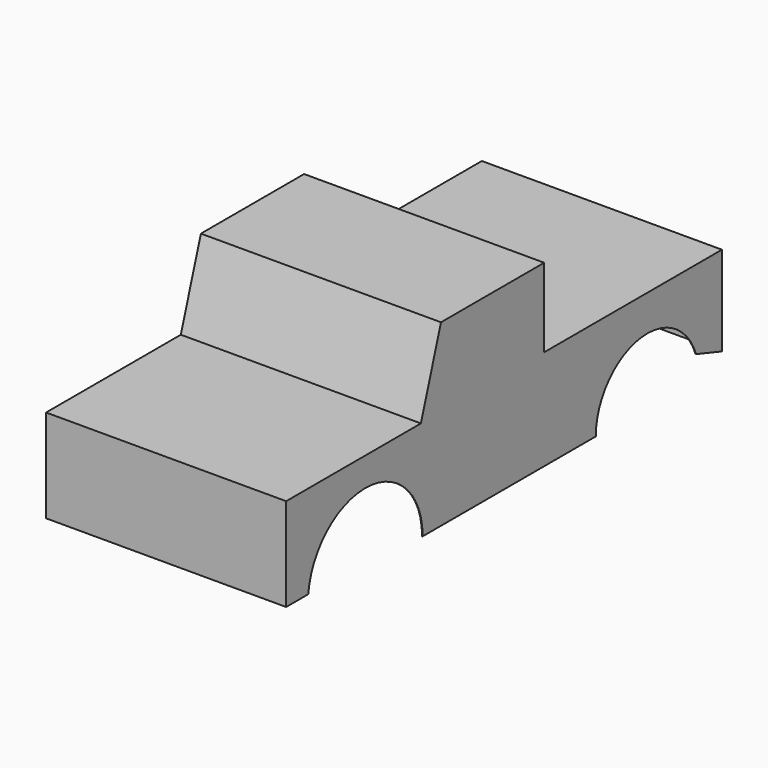
from build123d import *

# Parameters (mm, degrees)
F1_DEPTH = 106.3625
F2_T     = -0.508


with BuildPart() as f1:
    # F0 (on Right) → F1 (new body, symmetric)
    with BuildSketch(Plane.YZ):
        with BuildLine():
            ThreePointArc((-218.7567022563, 6.35), (-152.3960137837, 63.4203756425), (-92.075, 0))
            Line((-92.075, 0), (0, 0))
            Line((0, 0), (99.695, 0))
            ThreePointArc((99.695, 0), (147.1808219158, 56.3269576842), (210.7265367264, 19.05))
            Line((210.7265367264, 19.05), (239.395, 9.525))
            Line((239.395, 9.525), (239.395, 88.9))
            Line((239.395, 88.9), (42.545, 88.9))
            Line((42.545, 88.9), (42.545, 158.75))
            Line((42.545, 158.75), (-71.755, 158.75))
            Line((-71.755, 158.75), (-93.98, 88.9))
            Line((-93.98, 88.9), (-243.205, 88.9))
            Line((-243.205, 88.9), (-243.205, 6.35))
            Line((-243.205, 6.35), (-218.7567022563, 6.35))
        make_face()
    extrude(amount=F1_DEPTH, both=True)

    # F2
    f2_openings = [f1.faces().sort_by_distance(p)[0] for p in [
        (0, 3.81, 0),
        (0, 147.180822, 56.326958),
        (0, 225.060768, 14.2875),
        (0, -152.396014, 63.420376),
        (0, -230.980851, 6.35),
    ]]
    offset(amount=F2_T, openings=f2_openings, kind=Kind.INTERSECTION)


solid = f1.part
